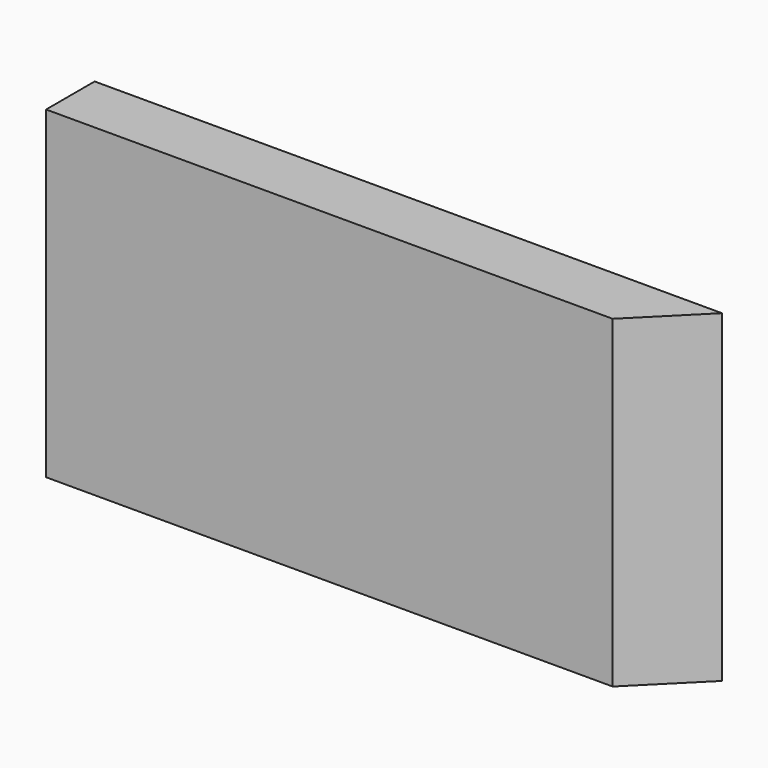
from build123d import *

# Parameters (mm, degrees)
F0_W     = 19.05
F0_H     = 101.6
F1_DEPTH = 19.05
F2_DEPTH = 196.85
F3_SIZE  = 19.04999


# Not quite as in the source:
# - a fillet or chamfer is up to 0.001 mm smaller than in the source, because OpenCascade refuses the exact size


with BuildPart() as f1:
    # F0 (on Right) → F1 (new body)
    with BuildSketch(Plane.YZ):
        Rectangle(F0_W, F0_H)
    extrude(amount=F1_DEPTH)

    # F0 (on Right) → F2 (join)
    with BuildSketch(Plane.YZ):
        Rectangle(F0_W, F0_H)
    extrude(amount=F2_DEPTH)

    # F3 (size 19.05 in the source; OpenCascade refuses exactly that, so slightly less here)
    f3_edges = [f1.edges().sort_by_distance(p)[0] for p in [
        (196.85, -9.525, 0),
    ]]
    chamfer(f3_edges, length=F3_SIZE)


solid = f1.part
